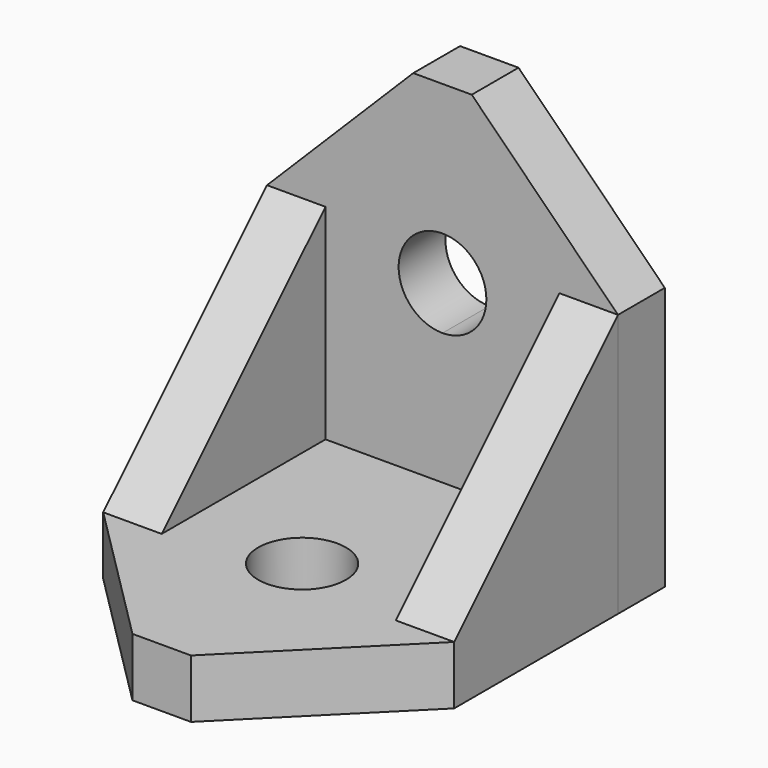
from build123d import *

# Parameters (mm, degrees)
F0_W     = 24
F0_H     = 24
F0_R     = 3
F1_DEPTH = 4
F3_DEPTH = 28
F5_DEPTH = 25
F6_SIZE  = 10
F7_W     = 4
F7_H     = 14
F8_DEPTH = 14
F9_SIZE  = 13.99999


# Not quite as in the source:
# - a fillet or chamfer is up to 0.001 mm smaller than in the source, because OpenCascade refuses the exact size


with BuildPart() as f1:
    # F0 (on Top) → F1 (new body)
    with BuildSketch(Plane.XY):
        Rectangle(F0_W, F0_H)
        Circle(F0_R, mode=Mode.SUBTRACT)
    extrude(amount=F1_DEPTH)

    # F2 (on Top) → F3 (join)
    with BuildSketch(Plane.XY):
        Polygon((-12.0000001043, 12), (0, 12), (11.9999998957, 12), (11.9999998957, 16), (-12.0000001043, 16), align=None)
    extrude(amount=F3_DEPTH)

    # F4 (on face) → F5 (cut)
    with BuildSketch(Plane.XZ.offset(-12)):
        with BuildLine():
            ThreePointArc((0, 13), (2.1213203436, 13.8786796564), (3, 16))
            ThreePointArc((3, 16), (-2.1213203436, 18.1213203436), (0, 13))
        make_face()
    extrude(amount=-F5_DEPTH, mode=Mode.SUBTRACT)

    # F6
    f6_edges = [f1.edges().sort_by_distance(p)[0] for p in [
        (-12, -12, 2),
        (12, -12, 2),
        (-12, 14, 28),
        (12, 14, 28),
    ]]
    chamfer(f6_edges, length=F6_SIZE)

    # F7 (on face) → F8 (join)
    with BuildSketch(Plane.XY.offset(4)):
        with Locations((-10, 5)):
            Rectangle(F7_W, F7_H)
        with Locations((10, 5)):
            Rectangle(F7_W, F7_H)
    extrude(amount=F8_DEPTH)

    # F9 (size 14 in the source; OpenCascade refuses exactly that, so slightly less here)
    f9_edges = [f1.edges().sort_by_distance(p)[0] for p in [
        (-10, -2, 18),
        (10, -2, 18),
    ]]
    chamfer(f9_edges, length=F9_SIZE)


solid = f1.part
